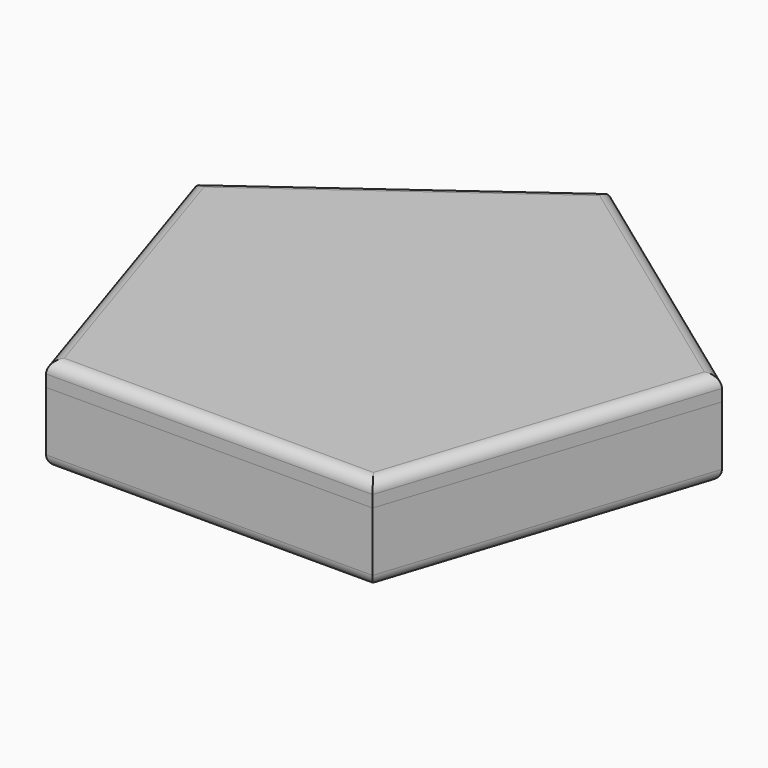
from build123d import *

# Parameters (mm, degrees)
F0_R     = 9.525
F0_R_2   = 31.75
F0_R_3   = 12.7
F0_R_4   = 4.7625
F1_DEPTH = 19.05
F2_DEPTH = 13.97
F3_DEPTH = 9.525
F4_R     = 1.5875
F5_R     = 3.175
F7_DEPTH = 6.35
F8_R     = 3.175


# Not quite as in the source:
# - a feature names something its author has since deleted; it is built from what else it names


with BuildPart() as f1:
    # F0 (on Top) → F1 (new body)
    with BuildSketch(Plane.XY):
        Polygon((-43.700125975, -60.1480633142), (43.700125975, -60.1480633142), (70.7082891401, 22.9745158286), (0, 74.3470949714), (-70.7082891401, 22.9745158286), align=None)
        with Locations((-29.8594908165, -41.0980633142)):
            Circle(F0_R, mode=Mode.SUBTRACT)
        with Locations((29.8594908165, -41.0980633142)):
            Circle(F0_R, mode=Mode.SUBTRACT)
        Circle(F0_R_2, mode=Mode.SUBTRACT)
        with Locations((-48.3136710278, 15.6980633142)):
            Circle(F0_R_3, mode=Mode.SUBTRACT)
        with Locations((-27.0081631652, 37.1735474857)):
            Circle(F0_R_4, mode=Mode.SUBTRACT)
        with Locations((27.0081631652, 37.1735474857)):
            Circle(F0_R_4, mode=Mode.SUBTRACT)
        with Locations((48.3136710278, 15.6980633142)):
            Circle(F0_R_3, mode=Mode.SUBTRACT)
        with Locations((0, 50.8)):
            Circle(F0_R_3, mode=Mode.SUBTRACT)
    extrude(amount=F1_DEPTH)

    # F0 (on Top) → F2 (join)
    with BuildSketch(Plane.XY):
        with Locations((-48.3136710278, 15.6980633142)):
            Circle(F0_R_3)
        with Locations((0, 50.8)):
            Circle(F0_R_3)
        with Locations((48.3136710278, 15.6980633142)):
            Circle(F0_R_3)
        with Locations((29.8594908165, -41.0980633142)):
            Circle(F0_R)
        with Locations((-29.8594908165, -41.0980633142)):
            Circle(F0_R)
        with Locations((-27.0081631652, 37.1735474857)):
            Circle(F0_R_4)
        with Locations((27.0081631652, 37.1735474857)):
            Circle(F0_R_4)
    extrude(amount=F2_DEPTH)

    # F0 (on Top) → F3 (join)
    with BuildSketch(Plane.XY):
        Circle(F0_R_2)
    extrude(amount=F3_DEPTH)

    # F4
    f4_edges = [f1.edges().sort_by_distance(p)[0] for p in [
        (-31.75, 0, 19.05),
    ]]
    fillet(f4_edges, radius=F4_R)

    # F5
    f5_edges = [f1.edges().sort_by_distance(p)[0] for p in [
        (0, -60.148063, 0),
        (57.204208, -18.586774, 0),
        (35.354145, 48.660805, 0),
        (-35.354145, 48.660805, 0),
        (-57.204208, -18.586774, 0),
    ]]
    fillet(f5_edges, radius=F5_R)


with BuildPart() as f7:
    # F6 (on face) → F7 (new body)
    with BuildSketch(Plane.XY.offset(19.05)):
        Polygon((-70.7082891401, 22.9745158286), (-43.700125975, -60.1480633142), (43.700125975, -60.1480633142), (70.7082891401, 22.9745158286), (0, 74.3470949714), align=None)
    extrude(amount=F7_DEPTH)

    # F8
    f8_edges = [f7.edges().sort_by_distance(p)[0] for p in [
        (-57.204208, -18.586774, 25.4),
        (0, -60.148063, 25.4),
        (57.204208, -18.586774, 25.4),
        (35.354145, 48.660805, 25.4),
        (-35.354145, 48.660805, 25.4),
    ]]
    fillet(f8_edges, radius=F8_R)


solid = Compound([f1.part, f7.part])
